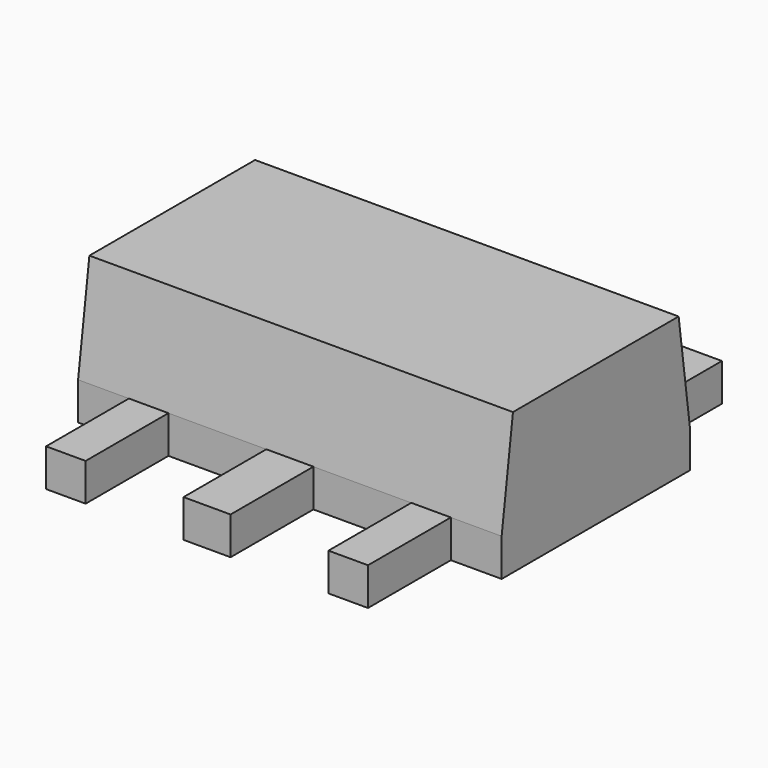
from build123d import *

# Parameters (mm, degrees)
F4_W       = 1.6
F4_H       = 1
F4_W_2     = 0.42
F4_H_2     = 0.5
F4_H_3     = 1.1
F4_W_3     = 0.5
F5_DEPTH   = 0.4
F6_DEPTH   = 0.2
F7_R       = 0.2
F4_W_4     = 0.49
F8_DEPTH   = 1.5
F9_SIZE2   = 0.15
F9_SIZE    = 1.1
F9_2_SIZE2 = 0.15
F9_2_SIZE  = 1.1
F10_DEPTH  = 0.4


with BuildPart() as f5:
    # F4 (on Top) → F5 (new body)
    with BuildSketch(Plane.XY):
        with Locations((0, 0.75)):
            Rectangle(F4_W, F4_H)
        Polygon((-1.29, -0.25), (-0.55, -0.25), (-0.8, 0), (-0.8, 0.25), (-1.29, 0.25), align=None)
        Polygon((-0.55, -0.25), (0.55, -0.25), (0.8, 0), (0.8, 0.25), (-0.8, 0.25), (-0.8, 0), align=None)
        Polygon((-0.25, -1.25), (0.25, -1.25), (0.25, -0.55), (0.55, -0.25), (-0.55, -0.25), (-0.25, -0.55), align=None)
        with Locations((-1.5, 0)):
            Rectangle(F4_W_2, F4_H_2)
        with Locations((-1.5, 0.75)):
            Rectangle(F4_W_2, F4_H)
        with Locations((-1.5, -0.75)):
            Rectangle(F4_W_2, F4_H)
        with Locations((-1.5, -1.8)):
            Rectangle(F4_W_2, F4_H_3)
        with Locations((0, -1.8)):
            Rectangle(F4_W_3, F4_H_3)
        Polygon((0.55, -0.25), (1.29, -0.25), (1.29, 0.25), (0.8, 0.25), (0.8, 0), align=None)
        with Locations((1.5, -0.75)):
            Rectangle(F4_W_2, F4_H)
        with Locations((1.5, -1.8)):
            Rectangle(F4_W_2, F4_H_3)
        with Locations((1.5, 0)):
            Rectangle(F4_W_2, F4_H_2)
        with Locations((1.5, 0.75)):
            Rectangle(F4_W_2, F4_H)
        with Locations((1.5, 1.8)):
            Rectangle(F4_W_2, F4_H_3)
        Polygon((-0.8, 1.25), (0.8, 1.25), (0.8, 1.8), (0.2, 1.8), (0.2, 2.35), (-0.2, 2.35), (-0.2, 1.8), (-0.8, 1.8), align=None)
        with Locations((-1.5, 1.8)):
            Rectangle(F4_W_2, F4_H_3)
    extrude(amount=F5_DEPTH)

    # F4 (on Top) → F6 (cut)
    with BuildSketch(Plane.XY):
        with Locations((-1.5, -0.75)):
            Rectangle(F4_W_2, F4_H)
        with Locations((-1.5, 0)):
            Rectangle(F4_W_2, F4_H_2)
        with Locations((-1.5, 0.75)):
            Rectangle(F4_W_2, F4_H)
        Polygon((-1.29, -0.25), (-0.55, -0.25), (-0.8, 0), (-0.8, 0.25), (-1.29, 0.25), align=None)
        Polygon((0.55, -0.25), (1.29, -0.25), (1.29, 0.25), (0.8, 0.25), (0.8, 0), align=None)
        with Locations((1.5, -0.75)):
            Rectangle(F4_W_2, F4_H)
        with Locations((1.5, 0)):
            Rectangle(F4_W_2, F4_H_2)
        with Locations((1.5, 0.75)):
            Rectangle(F4_W_2, F4_H)
    extrude(amount=F6_DEPTH, mode=Mode.SUBTRACT)

    # F7
    f7_edges = [f5.edges().sort_by_distance(p)[0] for p in [
        (-0.8, 1.8, 0.2),
        (-0.2, 1.8, 0.2),
        (0.2, 1.8, 0.2),
        (0.8, 1.8, 0.2),
    ]]
    fillet(f7_edges, radius=F7_R)


with BuildPart() as f8:
    # F4 (on Top) → F8 (new body)
    with BuildSketch(Plane.XY):
        Polygon((-1.29, -1.25), (-0.25, -1.25), (-0.25, -0.55), (-0.55, -0.25), (-1.29, -0.25), align=None)
        with Locations((-1.5, -0.75)):
            Rectangle(F4_W_2, F4_H)
        with Locations((-1.5, 0)):
            Rectangle(F4_W_2, F4_H_2)
        with Locations((-1.5, 0.75)):
            Rectangle(F4_W_2, F4_H)
        with Locations((-1.045, 0.75)):
            Rectangle(F4_W_4, F4_H)
        with Locations((0, 0.75)):
            Rectangle(F4_W, F4_H)
        Polygon((-1.29, -0.25), (-0.55, -0.25), (-0.8, 0), (-0.8, 0.25), (-1.29, 0.25), align=None)
        Polygon((-0.25, -1.25), (0.25, -1.25), (0.25, -0.55), (0.55, -0.25), (-0.55, -0.25), (-0.25, -0.55), align=None)
        Polygon((-0.55, -0.25), (0.55, -0.25), (0.8, 0), (0.8, 0.25), (-0.8, 0.25), (-0.8, 0), align=None)
        Polygon((0.25, -1.25), (1.29, -1.25), (1.29, -0.25), (0.55, -0.25), (0.25, -0.55), align=None)
        with Locations((1.5, -0.75)):
            Rectangle(F4_W_2, F4_H)
        Polygon((0.55, -0.25), (1.29, -0.25), (1.29, 0.25), (0.8, 0.25), (0.8, 0), align=None)
        with Locations((1.5, 0)):
            Rectangle(F4_W_2, F4_H_2)
        Polygon((1.71, -1.25), (2.25, -1.25), (2.25, 1.25), (1.71, 1.25), (1.71, 0.25), (1.71, -0.25), align=None)
        with Locations((1.045, 0.75)):
            Rectangle(F4_W_4, F4_H)
        with Locations((1.5, 0.75)):
            Rectangle(F4_W_2, F4_H)
        Polygon((-2.25, -1.25), (-1.71, -1.25), (-1.71, -0.25), (-1.71, 0.25), (-1.71, 1.25), (-2.25, 1.25), align=None)
    extrude(amount=F8_DEPTH)

    # F9
    f9_edges = [f8.edges().sort_by_distance(p)[0] for p in [
        (0, -1.25, 1.5),
    ]]
    f9_side = f8.faces().sort_by_distance((0, -1.25, 0.75))[0]
    chamfer(f9_edges, length=F9_SIZE, length2=F9_SIZE2, reference=f9_side)

    # F9#2
    f9_2_edges = [f8.edges().sort_by_distance(p)[0] for p in [
        (0, 1.25, 1.5),
    ]]
    f9_2_side = f8.faces().sort_by_distance((0, 1.25, 0.75))[0]
    chamfer(f9_2_edges, length=F9_2_SIZE, length2=F9_2_SIZE2, reference=f9_2_side)

    # F4 (on Top) → F10 (cut)
    with BuildSketch(Plane.XY):
        Polygon((-0.55, -0.25), (0.55, -0.25), (0.8, 0), (0.8, 0.25), (-0.8, 0.25), (-0.8, 0), align=None)
        Polygon((-0.25, -1.25), (0.25, -1.25), (0.25, -0.55), (0.55, -0.25), (-0.55, -0.25), (-0.25, -0.55), align=None)
        with Locations((0, 0.75)):
            Rectangle(F4_W, F4_H)
    extrude(amount=F10_DEPTH, mode=Mode.SUBTRACT)


solid = Compound([f5.part, f8.part])
